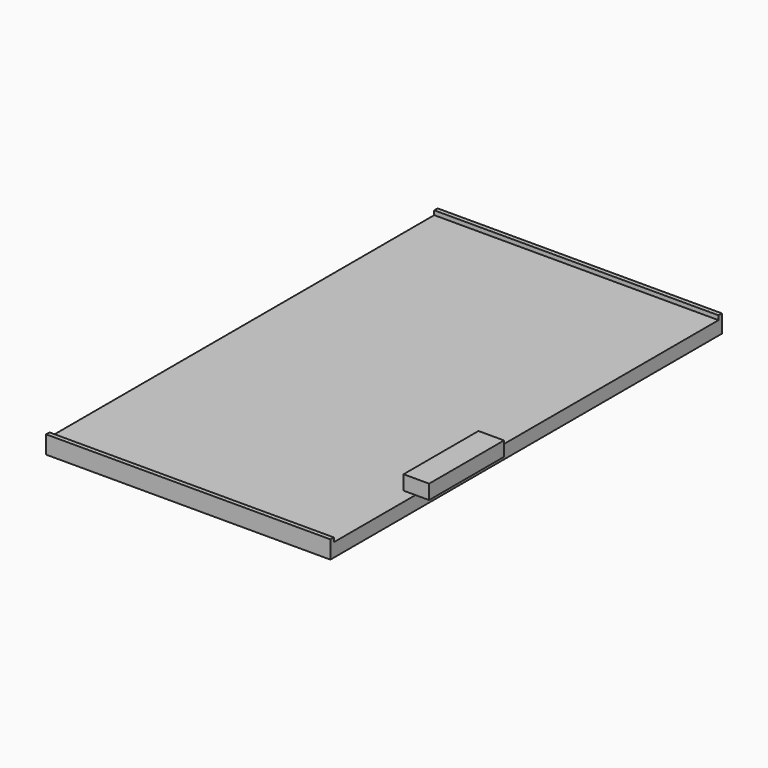
from build123d import *

# Parameters (mm, degrees)
F0_W     = 3500
F0_H     = 5750
F1_DEPTH = 160
F2_W     = 300
F2_H     = 1100
F3_DEPTH = 170
F4_W     = 160
F4_H     = 160
F5_DEPTH = 5750.001
F8_W     = 3340
F8_H     = 50
F9_DEPTH = 50


# Not quite as in the source:
# - a feature of the source that left no trace in its solid (it failed there, or was rolled back) is left out


with BuildPart() as f1:
    # F0 (on Top) → F1 (new body)
    with BuildSketch(Plane.XY):
        with Locations((1750, 2875)):
            Rectangle(F0_W, F0_H)
    extrude(amount=F1_DEPTH)

    # F2 (on face) → F3 (join)
    with BuildSketch(Plane.XY.offset(160)):
        with Locations((3350, 1800)):
            Rectangle(F2_W, F2_H)
    extrude(amount=F3_DEPTH)

    # F4 (on face) → F5 (cut, through all)
    with BuildSketch(Plane.XZ):
        with Locations((3420, 80)):
            Rectangle(F4_W, F4_H)
    extrude(amount=-F5_DEPTH, mode=Mode.SUBTRACT)

    # F8 (on face) → F9 (join)
    with BuildSketch(Plane.XY.offset(160)):
        with Locations((1670, 25)):
            Rectangle(F8_W, F8_H)
        with Locations((1670, 5725)):
            Rectangle(F8_W, F8_H)
    extrude(amount=F9_DEPTH)


solid = f1.part
